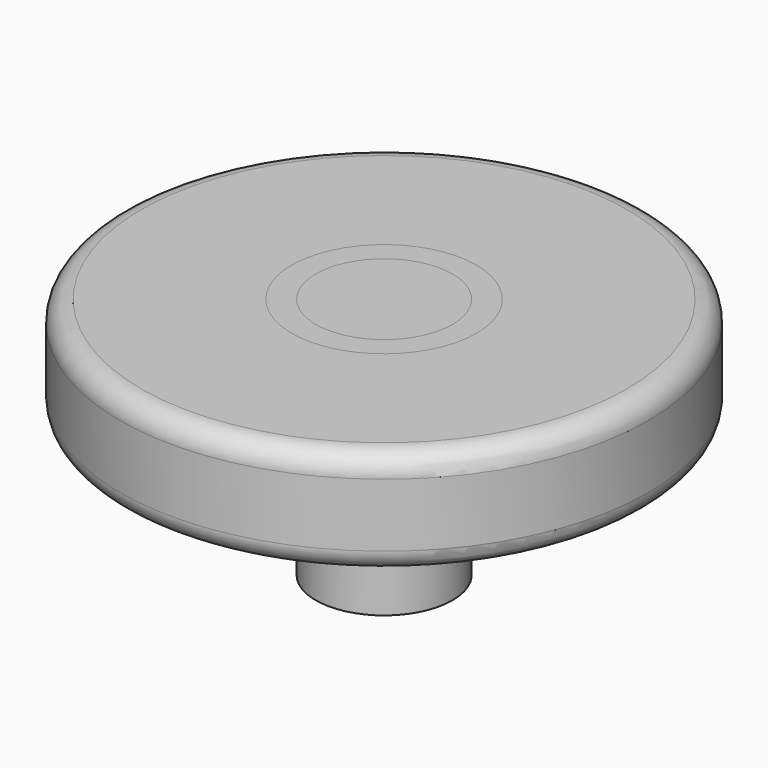
from build123d import *

# Parameters (mm, degrees)
F0_R     = 5
F0_R_2   = 1.75
F1_DEPTH = 2
F0_R_3   = 1.295
F3_DEPTH = 2
F4_DEPTH = 0.4
F5_DEPTH = 2
F6_R     = 0.4
F7_DEPTH = 2.6


# Not quite as in the source:
# - the program builds the solid bodies; features that only make, move or delete a surface that nothing else refers to are left out


with BuildPart() as f1:
    # F0 (on Top) → F1 (new body)
    with BuildSketch(Plane.XY):
        Circle(F0_R)
        Circle(F0_R_2, mode=Mode.SUBTRACT)
    extrude(amount=F1_DEPTH)

    # F6
    f6_edges = [f1.edges().sort_by_distance(p)[0] for p in [
        (-5, 0, 2),
        (-5, 0, 0),
    ]]
    fillet(f6_edges, radius=F6_R)


with BuildPart() as f3:
    # F0 (on Top) → F3 (new body)
    with BuildSketch(Plane.XY):
        Circle(F0_R_3)
    extrude(amount=F3_DEPTH)


with BuildPart() as f4:
    # F0 (on Top) → F4 (new body)
    with BuildSketch(Plane.XY):
        Circle(F0_R_2)
        Circle(F0_R_3, mode=Mode.SUBTRACT)
    extrude(amount=-F4_DEPTH)


with BuildPart() as f5:
    # F0 (on Top) → F5 (new body)
    with BuildSketch(Plane.XY):
        Circle(F0_R_2)
        Circle(F0_R_3, mode=Mode.SUBTRACT)
    extrude(amount=F5_DEPTH)


with BuildPart() as f7:
    # F7 (new): a face of the model
    f7_faces = [f3.part.faces().sort_by_distance(p)[0] for p in [
        (0, 0, 0),
    ]]
    extrude(f7_faces, amount=F7_DEPTH)


solid = Compound([f1.part, f3.part, f4.part, f5.part, f7.part])
